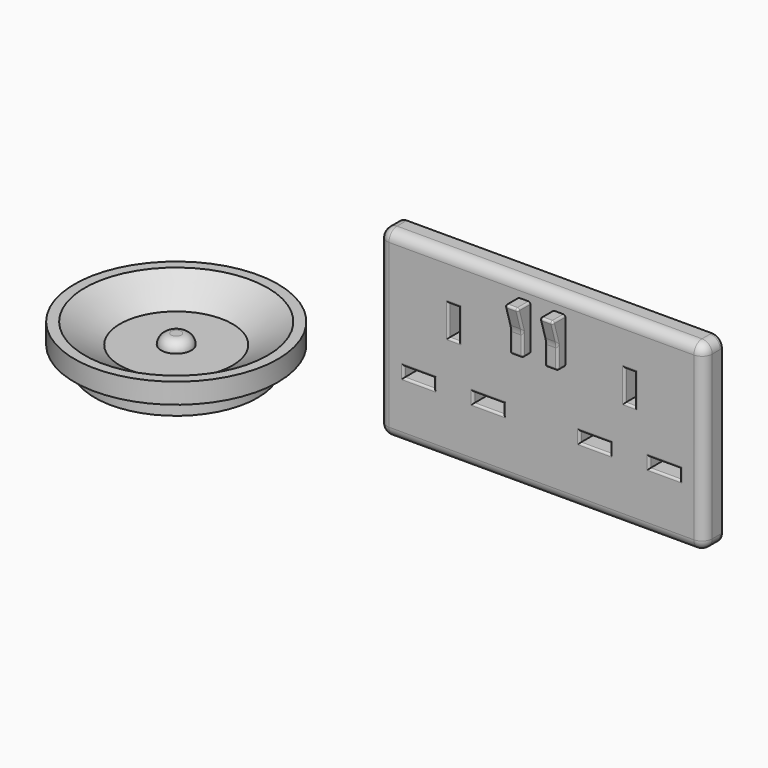
from build123d import *

# Parameters (mm, degrees)
F0_R      = 50
F1_DEPTH  = 10
F2_R      = 40
F3_DEPTH  = 10
F4_R      = 45
F5_DEPTH  = 10
F5_TAPER  = 60
F6_R      = 7.5
F7_DEPTH  = 5
F8_R      = 4.99999
F9_W      = 160
F9_H      = 90
F10_DEPTH = 10
F11_W     = 5
F11_H     = 15
F11_W_2   = 15
F11_H_2   = 5
F12_DEPTH = 15
F13_W     = 6.3590165973
F13_H     = 22.4987007678
F14_DEPTH = 8
F16_DEPTH = 25
F17_R     = 1
F18_R     = 10
F19_R     = 1
F20_R     = 5
F22_DEPTH = 1


# Not quite as in the source:
# - a fillet or chamfer is up to 0.001 mm smaller than in the source, because OpenCascade refuses the exact size


with BuildPart() as f1:
    # F0 (on Top) → F1 (new body)
    with BuildSketch(Plane.XY):
        Circle(F0_R)
    extrude(amount=F1_DEPTH)

    # F2 (on face) → F3 (join)
    with BuildSketch(Plane(origin=(0, 0, 0), x_dir=(1, 0, 0), z_dir=(0, 0, -1))):
        Circle(F2_R)
    extrude(amount=F3_DEPTH)

    # F4 (on face) → F5 (cut)
    with BuildSketch(Plane.XY.offset(10)):
        Circle(F4_R)
    extrude(amount=-F5_DEPTH, taper=F5_TAPER, mode=Mode.SUBTRACT)

    # F6 (on face) → F7 (join)
    with BuildSketch(Plane.XY):
        Circle(F6_R)
    extrude(amount=F7_DEPTH)

    # F8 (radius 5 in the source; OpenCascade refuses exactly that, so slightly less here)
    f8_edges = [f1.edges().sort_by_distance(p)[0] for p in [
        (-7.5, 0, 5),
    ]]
    fillet(f8_edges, radius=F8_R)


with BuildPart() as f10:
    # F9 (on Front) → F10 (new body)
    with BuildSketch(Plane.XZ):
        with Locations((187.6312586665, 45)):
            Rectangle(F9_W, F9_H)
    extrude(amount=F10_DEPTH)

    # F11 (on Front) → F12 (cut)
    with BuildSketch(Plane.XZ):
        with Locations((144.4571614265, 60.6002969737)):
            Rectangle(F11_W, F11_H)
        with Locations((127.3545090962, 31.1194501932)):
            Rectangle(F11_W_2, F11_H_2)
        with Locations((161.5598137569, 31.1194501932)):
            Rectangle(F11_W_2, F11_H_2)
        with Locations((231.0760170221, 60.6002969737)):
            Rectangle(F11_W, F11_H)
        with Locations((213.9733646918, 31.1194501932)):
            Rectangle(F11_W_2, F11_H_2)
        with Locations((248.1786693525, 31.1194501932)):
            Rectangle(F11_W_2, F11_H_2)
    extrude(amount=F12_DEPTH, mode=Mode.SUBTRACT)

    # F13 (on face) → F14 (join)
    with BuildSketch(Plane.XZ.offset(10)):
        with Locations((196.219098717, 70.5612506717)):
            Rectangle(F13_W, F13_H)
        with Locations((179.0434186161, 70.5612506717)):
            Rectangle(F13_W, F13_H)
    extrude(amount=F14_DEPTH)

    # F15 (on face) → F16 (cut)
    with BuildSketch(Plane.YZ.offset(199.3986070156)):
        Polygon((-14.6644348279, 59.3119002879), (-14.6644348279, 70.5612506717), (-18, 81.8106010556), (-18, 59.3119002879), align=None)
    extrude(amount=-F16_DEPTH, mode=Mode.SUBTRACT)

    # F17
    f17_edges = [f10.edges().sort_by_distance(p)[0] for p in [
        (199.398607, -14.664435, 64.936575),
        (199.398607, -16.332217, 76.185926),
        (196.219099, -18, 81.810601),
        (179.043419, -18, 81.810601),
        (193.03959, -16.332217, 76.185926),
        (193.03959, -14.664435, 64.936575),
        (196.219099, -14.664435, 59.3119),
        (199.398607, -14, 81.810601),
        (199.398607, -12.332217, 59.3119),
        (193.03959, -12.332217, 59.3119),
        (193.03959, -14, 81.810601),
        (182.222927, -14.664435, 64.936575),
        (182.222927, -16.332217, 76.185926),
        (175.86391, -16.332217, 76.185926),
        (175.86391, -14.664435, 64.936575),
        (179.043419, -14.664435, 59.3119),
        (175.86391, -12.332217, 59.3119),
        (182.222927, -12.332217, 59.3119),
        (182.222927, -14, 81.810601),
        (175.86391, -14, 81.810601),
    ]]
    fillet(f17_edges, radius=F17_R)

    # F18
    f18_edges = [f10.edges().sort_by_distance(p)[0] for p in [
        (179.043419, -14.664435, 70.561251),
        (196.219099, -14.664435, 70.561251),
    ]]
    fillet(f18_edges, radius=F18_R)

    # F19
    f19_edges = [f10.edges().sort_by_distance(p)[0] for p in [
        (141.957161, -10, 60.600297),
        (144.457161, -10, 53.100297),
        (146.957161, -10, 60.600297),
        (144.457161, -10, 68.100297),
        (127.354509, -10, 33.61945),
        (119.854509, -10, 31.11945),
        (127.354509, -10, 28.61945),
        (134.854509, -10, 31.11945),
        (154.059814, -10, 31.11945),
        (161.559814, -10, 33.61945),
        (169.059814, -10, 31.11945),
        (161.559814, -10, 28.61945),
        (213.973365, -10, 28.61945),
        (213.973365, -10, 33.61945),
        (206.473365, -10, 31.11945),
        (221.473365, -10, 31.11945),
        (248.178669, -10, 33.61945),
        (240.678669, -10, 31.11945),
        (248.178669, -10, 28.61945),
        (255.678669, -10, 31.11945),
        (231.076017, -10, 68.100297),
        (228.576017, -10, 60.600297),
        (231.076017, -10, 53.100297),
        (233.576017, -10, 60.600297),
    ]]
    fillet(f19_edges, radius=F19_R)

    # F20
    f20_edges = [f10.edges().sort_by_distance(p)[0] for p in [
        (267.631259, -5, 90),
        (107.631259, -5, 90),
        (107.631259, -5, 0),
        (267.631259, -5, 0),
        (187.631259, -10, 90),
        (267.631259, -10, 45),
        (187.631259, -10, 0),
        (107.631259, -10, 45),
    ]]
    fillet(f20_edges, radius=F20_R)

    # F21 (on face) → F22 (join)
    with BuildSketch(Plane(origin=(0, 0, 0), x_dir=(-1, 0, 0), z_dir=(0, 1, 0))):
        with BuildLine():
            Line((-262.6312586665, 0), (-112.6312586665, 0))
            ThreePointArc((-112.6312586665, 0), (-109.0957247606, 1.4644660941), (-107.6312586665, 5))
            Line((-107.6312586665, 5), (-107.6312586665, 85))
            ThreePointArc((-107.6312586665, 85), (-109.0957247606, 88.5355339059), (-112.6312586665, 90))
            Line((-112.6312586665, 90), (-262.6312586665, 90))
            ThreePointArc((-262.6312586665, 90), (-266.1667925724, 88.5355339059), (-267.6312586665, 85))
            Line((-267.6312586665, 85), (-267.6312586665, 5))
            ThreePointArc((-267.6312586665, 5), (-266.1667925724, 1.4644660941), (-262.6312586665, 0))
        make_face()
    extrude(amount=F22_DEPTH)


solid = Compound([f1.part, f10.part])
